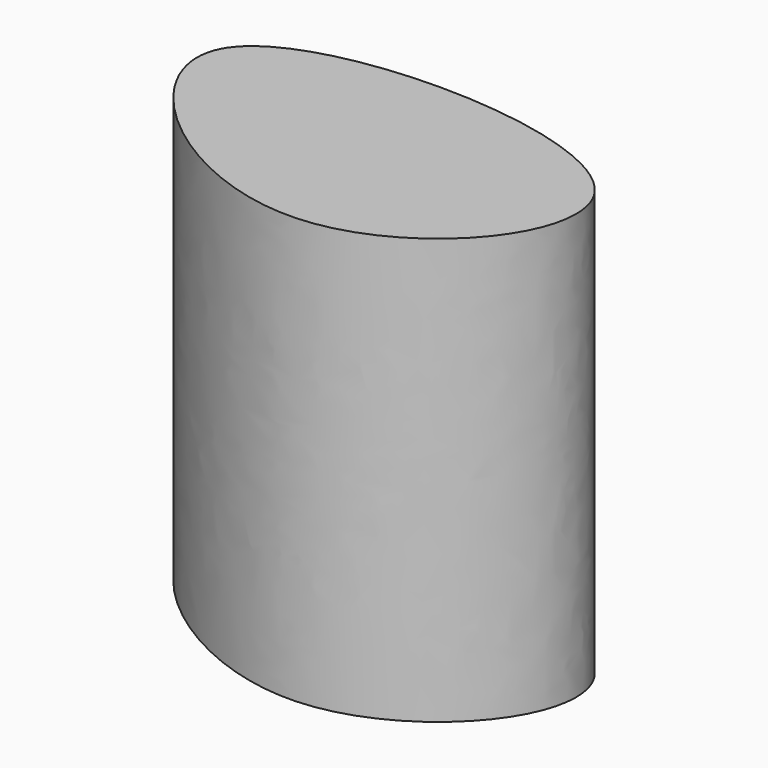
from build123d import *

# Parameters (mm, degrees)
F3_DEPTH = 25.4


# Not quite as in the source:
# - the program builds the solid bodies; features that only make, move or delete a surface that nothing else refers to are left out


with BuildPart() as f3:
    # F2 (on Top) → F3 (new body)
    with BuildSketch(Plane.XY):
        with BuildLine():
            add(Edge.make_bspline(
                [(22.5669257343, 24.8749051243), (19.1224438946, 29.6797083312), (-11.8993173459, 30.0820552908), (13.7441964683, 6.9436916311), (25.2975180775, 21.0659261667), (22.5669257343, 24.8749051243)],
                knots=[0, 0, 0, 0, 0.3741900355, 0.7033630911, 1, 1, 1, 1], degree=3))
        make_face()
    extrude(amount=-F3_DEPTH)


solid = f3.part
